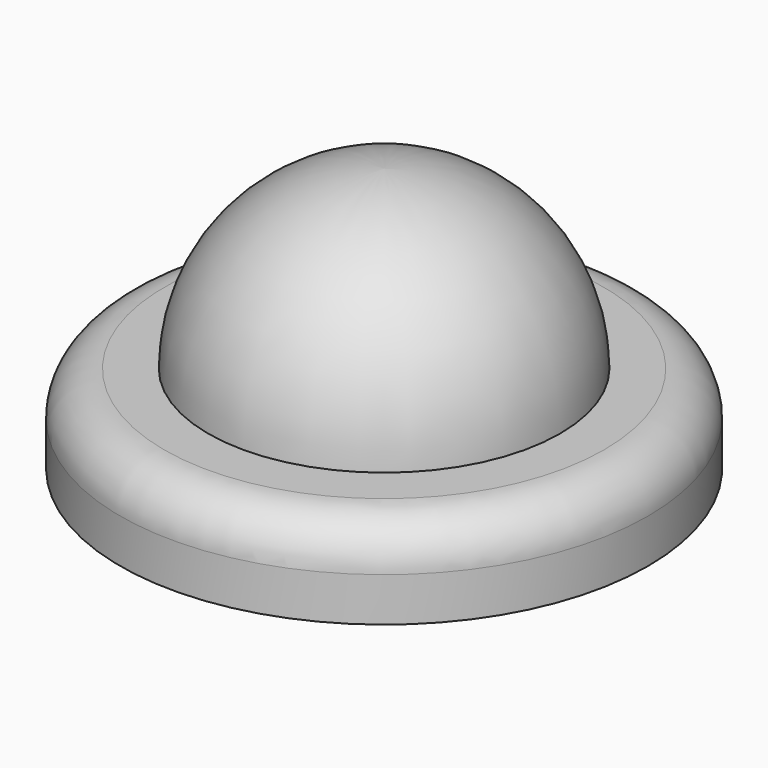
from build123d import *

# Parameters (mm, degrees)
F0_R     = 4
F1_DEPTH = 4
F2_R     = 3.99999
F3_R     = 6
F4_DEPTH = 2
F5_R     = 1


# Not quite as in the source:
# - a fillet or chamfer is up to 0.001 mm smaller than in the source, because OpenCascade refuses the exact size


with BuildPart() as f1:
    # F0 (on Top) → F1 (new body)
    with BuildSketch(Plane.XY):
        Circle(F0_R)
    extrude(amount=F1_DEPTH)

    # F2 (radius 4 in the source; OpenCascade refuses exactly that, so slightly less here)
    f2_edges = [f1.edges().sort_by_distance(p)[0] for p in [
        (-4, 0, 4),
    ]]
    fillet(f2_edges, radius=F2_R)


with BuildPart() as f4:
    # F3 (on Top) → F4 (new body)
    with BuildSketch(Plane.XY):
        Circle(F3_R)
    extrude(amount=-F4_DEPTH)

    # F5
    f5_edges = [f4.edges().sort_by_distance(p)[0] for p in [
        (-6, 0, 0),
    ]]
    fillet(f5_edges, radius=F5_R)


solid = Compound([f1.part, f4.part])
